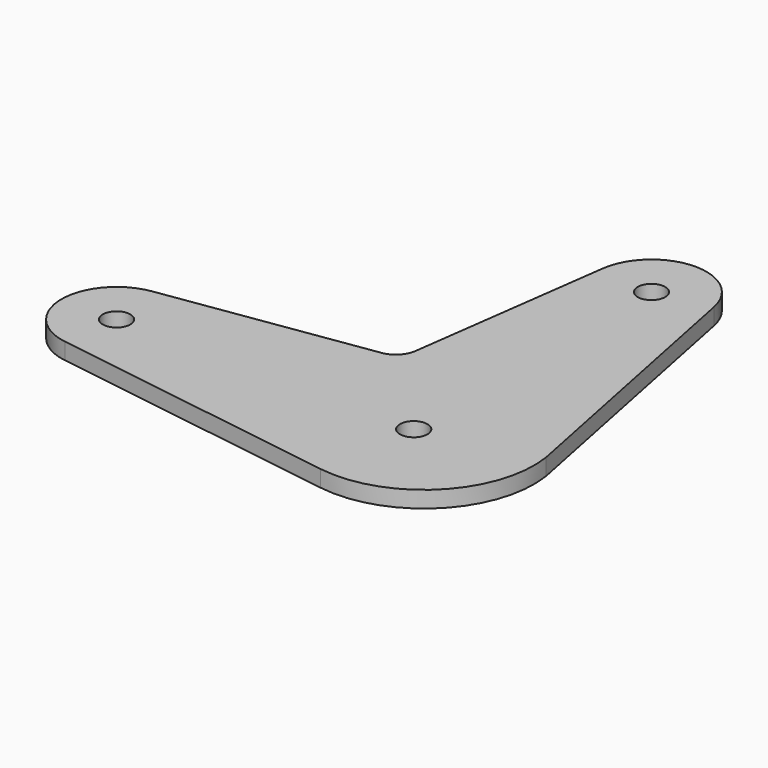
from build123d import *

# Parameters (mm, degrees)
F0_R     = 3.96875
F1_DEPTH = 4.7625
F2_R     = 6.35


# Not quite as in the source:
# - a feature names something its author has since deleted; it is built from what else it names


with BuildPart() as f1:
    # F0 (on Top) → F1 (new body)
    with BuildSketch(Plane.XY):
        with BuildLine():
            Line((31.8700148185, 7.8436681485), (15.5628504577, 88.8576204098))
            ThreePointArc((15.5628504577, 88.8576204098), (-0.5130479886, 101.5917074959), (-15.732715337, 87.8456822313))
            Line((-15.732715337, 87.8456822313), (-24.1670854724, 25.2735804658))
            Line((-24.1670854724, 25.2735804658), (-88.0768518519, 15.6998222241))
            ThreePointArc((-88.0768518519, 15.6998222241), (-101.6, 0), (-88.0768518519, -15.6998222241))
            Line((-88.0768518519, -15.6998222241), (-4.2333333333, -28.2596800033))
            ThreePointArc((-4.2333333333, -28.2596800033), (22.921010673, -19.3106758579), (31.8700148185, 7.8436681485))
        make_face()
        with Locations((-85.725, 0)):
            Circle(F0_R, mode=Mode.SUBTRACT)
        Circle(F0_R, mode=Mode.SUBTRACT)
        with Locations((0, 85.725)):
            Circle(F0_R, mode=Mode.SUBTRACT)
    extrude(amount=F1_DEPTH)

    # F2
    f2_edges = [f1.edges().sort_by_distance(p)[0] for p in [
        (-24.167085, 25.27358, 2.38125),
    ]]
    fillet(f2_edges, radius=F2_R)


solid = f1.part
